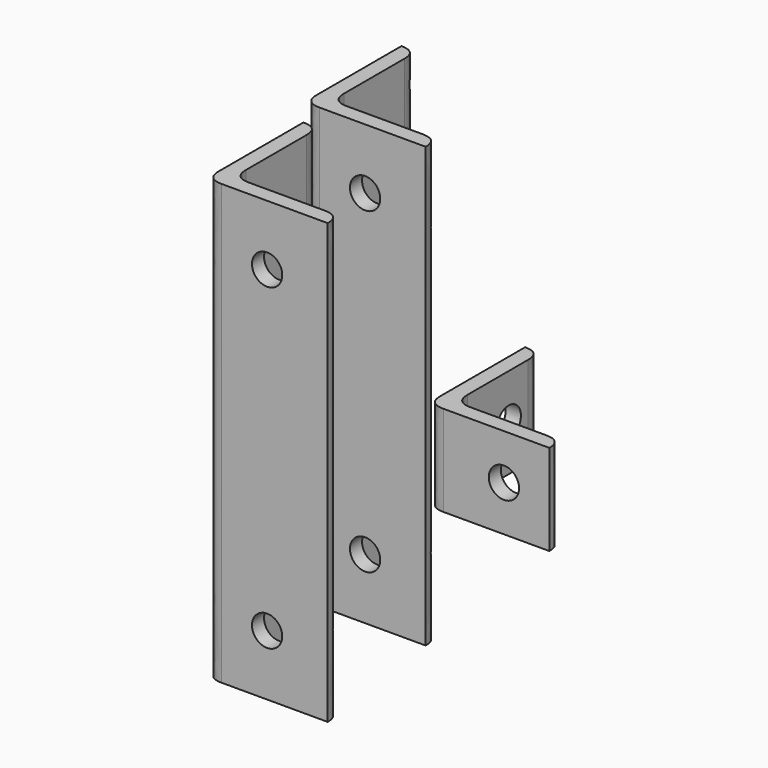
from build123d import *

# Parameters (mm, degrees)
F1_DEPTH       = 25.4
F3_DEPTH       = 92.075
F7_R           = 3.175
F9_DEPTH       = 3.175
F8_R           = 3.175
F10_DEPTH      = 3.175
F11_R          = 3.175
F13_DEPTH      = 3.175
F12_R          = 3.175
F14_DEPTH      = 3.175
F6_R           = 3.175
F15_DEPTH      = 3.175
F16_R          = 3.175
F17_DEPTH      = 3.175
F18_T1_DEPTH   = 92.075
F18_T3_DEPTH   = 107.95
F18_2_T1_DEPTH = 25.4
F18_2_T3_DEPTH = 41.275
F18_3_T1_DEPTH = 92.075
F18_3_T3_DEPTH = 107.95
F19_DEPTH      = 1.5875
F20_DEPTH      = 1.5875
F21_DEPTH      = 1.5875
F22_DEPTH      = 1.5875


# Not quite as in the source:
# - a fillet or chamfer that OpenCascade refuses, or shapes differently, is made with other operations: its cross-section is extruded or revolved along the edge and cut away or added


with BuildPart() as f1:
    # F0 (on Top) → F1 (new body)
    with BuildSketch(Plane.XY):
        Polygon((-35.3384790047, 29.2046858582), (-38.5134790047, 29.2046858582), (-38.5134790047, 3.8046858582), (-13.1134790047, 3.8046858582), (-13.1134790047, 6.9796858582), (-35.3384790047, 6.9796858582), align=None)
    extrude(amount=F1_DEPTH)

    # F6 (on face) → F15 (cut)
    with BuildSketch(Plane.YZ.offset(-35.3384790047)):
        with Locations((20.9496858582, 12.7)):
            Circle(F6_R)
    extrude(amount=-F15_DEPTH, mode=Mode.SUBTRACT)

    # F16 (on face) → F17 (cut)
    with BuildSketch(Plane(origin=(0, 6.9796858582, 0), x_dir=(-1, 0, 0), z_dir=(0, 1, 0))):
        with Locations((22.6384790047, 12.7)):
            Circle(F16_R)
    extrude(amount=-F17_DEPTH, mode=Mode.SUBTRACT)

    # F18#2: fillet of radius 3.175 on 4 edges, made by hand

    # F18_2_s2 → F18_2_t1 (join)
    with BuildSketch(Plane.XY):
        with BuildLine():
            add(Edge.make_bspline(
                [(-35.3384790047, 10.1546858582), (-35.3384790047, 6.9796858582), (-32.1634790047, 6.9796858582)],
                knots=[0, 0, 0, 1, 1, 1], degree=2, weights=[1, 1, 1]))
            Line((-32.1634790047, 6.9796858582), (-35.3384790047, 6.9796858582))
            Line((-35.3384790047, 6.9796858582), (-35.3384790047, 10.1546858582))
        make_face()
    extrude(amount=F18_2_T1_DEPTH)

    # F18_2_s4 → F18_2_t3 (cut)
    with BuildSketch(Plane.XY.offset(-7.9375)):
        with BuildLine():
            add(Edge.make_bspline(
                [(-38.5134790047, 6.9796858582), (-38.5134790047, 3.8046858582), (-35.3384790047, 3.8046858582)],
                knots=[0, 0, 0, 1, 1, 1], degree=2, weights=[1, 1, 1]))
            Line((-35.3384790047, 3.8046858582), (-38.5134790047, 3.8046858582))
            Line((-38.5134790047, 3.8046858582), (-38.5134790047, 6.9796858582))
        make_face()
        with BuildLine():
            add(Edge.make_bspline(
                [(-13.1134790047, 3.8046858582), (-13.1134790047, 6.9796858582), (-16.2884790047, 6.9796858582)],
                knots=[0, 0, 0, 1, 1, 1], degree=2, weights=[1, 1, 1]))
            Line((-16.2884790047, 6.9796858582), (-13.1134790047, 6.9796858582))
            Line((-13.1134790047, 6.9796858582), (-13.1134790047, 3.8046858582))
        make_face()
        with BuildLine():
            add(Edge.make_bspline(
                [(-38.5134790047, 29.2046858582), (-35.3384790047, 29.2046858582), (-35.3384790047, 26.0296858582)],
                knots=[0, 0, 0, 1, 1, 1], degree=2, weights=[1, 1, 1]))
            Line((-35.3384790047, 26.0296858582), (-35.3384790047, 29.2046858582))
            Line((-35.3384790047, 29.2046858582), (-38.5134790047, 29.2046858582))
        make_face()
    extrude(amount=F18_2_T3_DEPTH, mode=Mode.SUBTRACT)

    # F19 (cut): a face of the model
    f19_faces = [f1.faces().sort_by_distance(p)[0] for p in [
        (-36.3862356489, 28.1569424984, 0),
    ]]
    extrude(f19_faces, amount=-F19_DEPTH, mode=Mode.SUBTRACT)

    # F20 (cut): a face of the model
    f20_faces = [f1.faces().sort_by_distance(p)[0] for p in [
        (-36.3862356489, 28.1569424984, 25.4),
    ]]
    extrude(f20_faces, amount=-F20_DEPTH, mode=Mode.SUBTRACT)

    # F21 (cut): a face of the model
    f21_faces = [f1.faces().sort_by_distance(p)[0] for p in [
        (-36.3862356489, 28.1569424984, 1.5875),
    ]]
    extrude(f21_faces, amount=-F21_DEPTH, mode=Mode.SUBTRACT)

    # F22 (cut): a face of the model
    f22_faces = [f1.faces().sort_by_distance(p)[0] for p in [
        (-36.3862356489, 28.1569424984, 23.8125),
    ]]
    extrude(f22_faces, amount=-F22_DEPTH, mode=Mode.SUBTRACT)


with BuildPart() as f3:
    # F0 (on Top) → F3 (new body)
    with BuildSketch(Plane.XY):
        Polygon((4.3401528042, 29.2046858582), (4.3401528042, 3.8046858582), (29.7401528042, 3.8046858582), (29.7401528042, 6.9796858582), (7.5151528042, 6.9796858582), (7.5151528042, 29.2046858582), align=None)
    extrude(amount=F3_DEPTH)


with BuildPart() as f3b:
    # F2 (on Top) → F3, piece 2 (new body)
    with BuildSketch(Plane.XY):
        Polygon((-37.2105298044, -4.8463200888), (-37.2105298044, -30.2463200888), (-11.8105298044, -30.2463200888), (-11.8105298044, -27.0713200888), (-34.0355298044, -27.0713200888), (-34.0355298044, -4.8463200888), align=None)
    extrude(amount=F3_DEPTH)

    # F8 (on face) → F10 (cut)
    with BuildSketch(Plane(origin=(0, -27.0713200888, 0), x_dir=(-1, 0, 0), z_dir=(0, 1, 0))):
        with Locations((24.5105298044, 79.375)):
            Circle(F8_R)
        with Locations((24.5105298044, 12.7)):
            Circle(F8_R)
    extrude(amount=-F10_DEPTH, mode=Mode.SUBTRACT)

    # F12 (on face) → F14 (cut)
    with BuildSketch(Plane.YZ.offset(-34.0355298044)):
        with Locations((-17.5463200888, 79.375)):
            Circle(F12_R)
        with Locations((-17.5463200888, 12.7)):
            Circle(F12_R)
    extrude(amount=-F14_DEPTH, mode=Mode.SUBTRACT)

    # F18: fillet of radius 3.175 on 4 edges, made by hand

    # F18_s2 → F18_t1 (join)
    with BuildSketch(Plane.XY):
        with BuildLine():
            add(Edge.make_bspline(
                [(-34.0355298044, -23.8963200888), (-34.0355298044, -27.0713200888), (-30.8605298044, -27.0713200888)],
                knots=[0, 0, 0, 1, 1, 1], degree=2, weights=[1, 1, 1]))
            Line((-30.8605298044, -27.0713200888), (-34.0355298044, -27.0713200888))
            Line((-34.0355298044, -27.0713200888), (-34.0355298044, -23.8963200888))
        make_face()
    extrude(amount=F18_T1_DEPTH)

    # F18_s4 → F18_t3 (cut)
    with BuildSketch(Plane.XY.offset(-7.9375)):
        with BuildLine():
            add(Edge.make_bspline(
                [(-37.2105298044, -27.0713200888), (-37.2105298044, -30.2463200888), (-34.0355298044, -30.2463200888)],
                knots=[0, 0, 0, 1, 1, 1], degree=2, weights=[1, 1, 1]))
            Line((-34.0355298044, -30.2463200888), (-37.2105298044, -30.2463200888))
            Line((-37.2105298044, -30.2463200888), (-37.2105298044, -27.0713200888))
        make_face()
        with BuildLine():
            add(Edge.make_bspline(
                [(-11.8105298044, -30.2463200888), (-11.8105298044, -27.0713200888), (-14.9855298044, -27.0713200888)],
                knots=[0, 0, 0, 1, 1, 1], degree=2, weights=[1, 1, 1]))
            Line((-14.9855298044, -27.0713200888), (-11.8105298044, -27.0713200888))
            Line((-11.8105298044, -27.0713200888), (-11.8105298044, -30.2463200888))
        make_face()
        with BuildLine():
            add(Edge.make_bspline(
                [(-34.0355298044, -8.0213200888), (-34.0355298044, -4.8463200888), (-37.2105298044, -4.8463200888)],
                knots=[0, 0, 0, 1, 1, 1], degree=2, weights=[1, 1, 1]))
            Line((-37.2105298044, -4.8463200888), (-34.0355298044, -4.8463200888))
            Line((-34.0355298044, -4.8463200888), (-34.0355298044, -8.0213200888))
        make_face()
    extrude(amount=F18_T3_DEPTH, mode=Mode.SUBTRACT)


with BuildPart() as f3c:
    # F2 (on Top) → F3, piece 3 (new body)
    with BuildSketch(Plane.XY):
        Polygon((-7.4239719417, -4.8463200888), (-7.4239719417, -30.2463200888), (17.9760280583, -30.2463200888), (17.9760280583, -27.0713200888), (-4.2489719417, -27.0713200888), (-4.2489719417, -4.8463200888), align=None)
    extrude(amount=F3_DEPTH)


with BuildPart() as f3d:
    # F2 (on Top) → F3, piece 4 (new body)
    with BuildSketch(Plane.XY):
        Polygon((-32.8239719417, -36.0129921032), (-32.8239719417, -61.4129921032), (-7.4239719417, -61.4129921032), (-7.4239719417, -58.2379921032), (-29.6489719417, -58.2379921032), (-29.6489719417, -36.0129921032), align=None)
    extrude(amount=F3_DEPTH)

    # F7 (on face) → F9 (cut)
    with BuildSketch(Plane(origin=(0, -58.2379921032, 0), x_dir=(-1, 0, 0), z_dir=(0, 1, 0))):
        with Locations((20.1239719417, 79.375)):
            Circle(F7_R)
        with Locations((20.1239719417, 12.7)):
            Circle(F7_R)
    extrude(amount=-F9_DEPTH, mode=Mode.SUBTRACT)

    # F11 (on face) → F13 (cut)
    with BuildSketch(Plane.YZ.offset(-29.6489719417)):
        with Locations((-48.7129921032, 79.375)):
            Circle(F11_R)
        with Locations((-48.7129921032, 12.7)):
            Circle(F11_R)
    extrude(amount=-F13_DEPTH, mode=Mode.SUBTRACT)

    # F18#3: fillet of radius 3.175 on 4 edges, made by hand

    # F18_3_s2 → F18_3_t1 (join)
    with BuildSketch(Plane.XY):
        with BuildLine():
            add(Edge.make_bspline(
                [(-29.6489719417, -55.0629921032), (-29.6489719417, -58.2379921032), (-26.4739719417, -58.2379921032)],
                knots=[0, 0, 0, 1, 1, 1], degree=2, weights=[1, 1, 1]))
            Line((-26.4739719417, -58.2379921032), (-29.6489719417, -58.2379921032))
            Line((-29.6489719417, -58.2379921032), (-29.6489719417, -55.0629921032))
        make_face()
    extrude(amount=F18_3_T1_DEPTH)

    # F18_3_s4 → F18_3_t3 (cut)
    with BuildSketch(Plane.XY.offset(-7.9375)):
        with BuildLine():
            add(Edge.make_bspline(
                [(-32.8239719417, -58.2379921032), (-32.8239719417, -61.4129921032), (-29.6489719417, -61.4129921032)],
                knots=[0, 0, 0, 1, 1, 1], degree=2, weights=[1, 1, 1]))
            Line((-29.6489719417, -61.4129921032), (-32.8239719417, -61.4129921032))
            Line((-32.8239719417, -61.4129921032), (-32.8239719417, -58.2379921032))
        make_face()
        with BuildLine():
            add(Edge.make_bspline(
                [(-7.4239719417, -61.4129921032), (-7.4239719417, -58.2379921032), (-10.5989719417, -58.2379921032)],
                knots=[0, 0, 0, 1, 1, 1], degree=2, weights=[1, 1, 1]))
            Line((-10.5989719417, -58.2379921032), (-7.4239719417, -58.2379921032))
            Line((-7.4239719417, -58.2379921032), (-7.4239719417, -61.4129921032))
        make_face()
        with BuildLine():
            add(Edge.make_bspline(
                [(-32.8239719417, -36.0129921032), (-29.6489719417, -36.0129921032), (-29.6489719417, -39.1879921032)],
                knots=[0, 0, 0, 1, 1, 1], degree=2, weights=[1, 1, 1]))
            Line((-29.6489719417, -39.1879921032), (-29.6489719417, -36.0129921032))
            Line((-29.6489719417, -36.0129921032), (-32.8239719417, -36.0129921032))
        make_face()
    extrude(amount=F18_3_T3_DEPTH, mode=Mode.SUBTRACT)


solid = Compound([f1.part, f3b.part, f3d.part])
